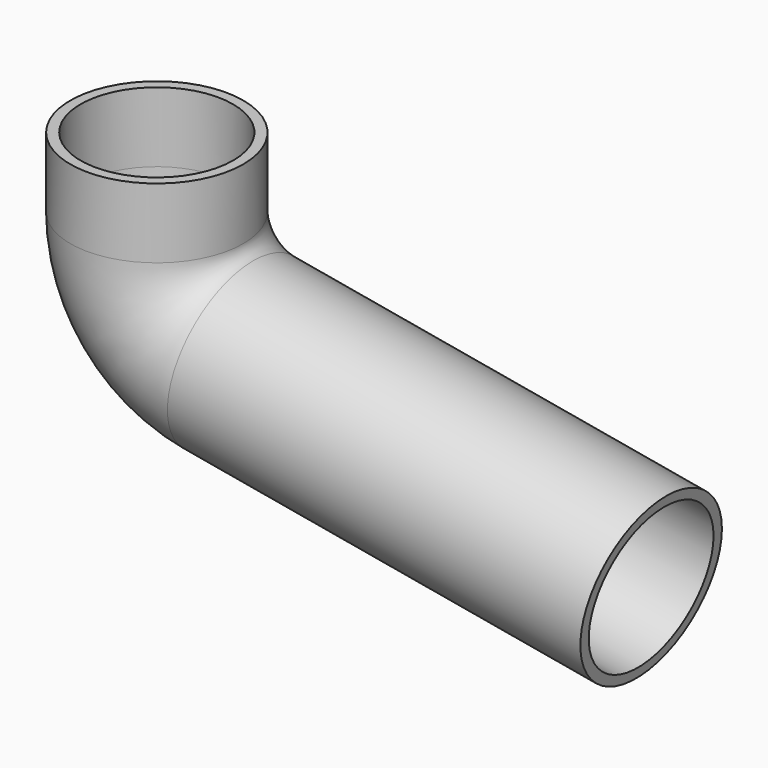
from build123d import *

# Parameters (mm, degrees)
F1_R   = 31.4265848645
F1_R_2 = 27.7125712081


# Not quite as in the source:
# - the program builds the solid bodies; features that only make, move or delete a surface that nothing else refers to are left out


with BuildPart() as f2:
    # F2: sweep along a path in F0
    with BuildLine(Plane.XZ) as f2_path:
        Line((-35.56, 25.4), (-35.56, 0))
        ThreePointArc((-35.56, 0), (-27.2405403973, -22.8575274005), (-6.1749291978, -35.0197636971))
        Line((-6.1749291978, -35.0197636971), (143.9097723612, -61.4837459736))
    # F1 (on Top) → F2 (sweep)
    with BuildSketch(Plane.XY):
        with Locations((-35.7853956521, 0)):
            Circle(F1_R)
        with Locations((-35.7853956521, 0)):
            Circle(F1_R_2, mode=Mode.SUBTRACT)
    sweep(path=f2_path.line)


solid = f2.part
